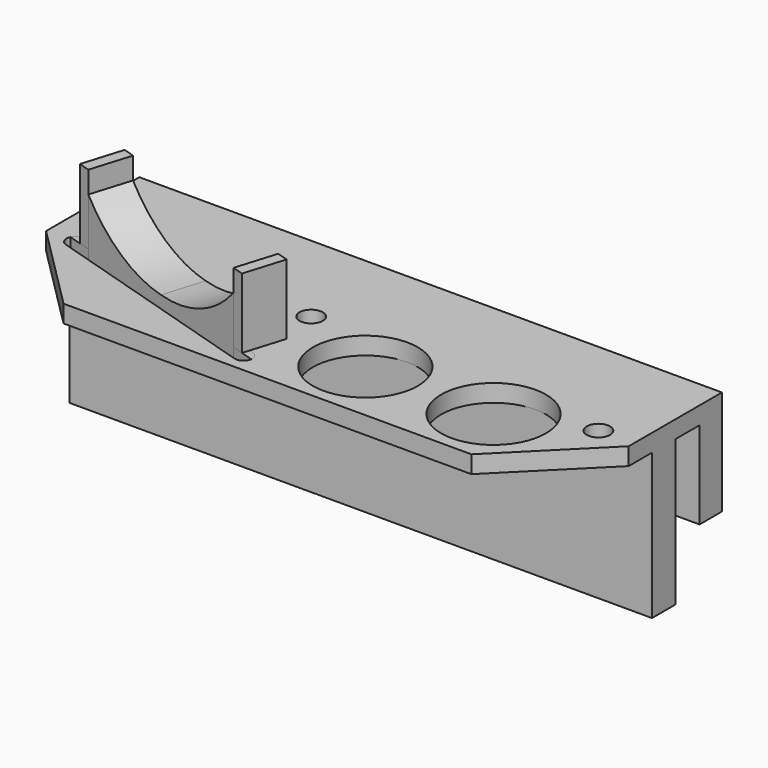
from build123d import *

# Parameters (mm, degrees)
F0_W      = 100
F0_H      = 35
F1_DEPTH  = 3
F2_W      = 100
F2_H      = 5
F3_DEPTH  = 25
F2_H_2    = 4.8
F4_DEPTH  = 15
F5_SIZE   = 15
F6_R      = 9
F6_R_2    = 2
F7_DEPTH  = 30
F9_DEPTH  = 1.25
F10_DEPTH = 6
F12_DEPTH = 3
F14_DEPTH = 12


with BuildPart() as f1:
    # F0 (on Top) → F1 (new body)
    with BuildSketch(Plane.XY):
        Rectangle(F0_W, F0_H)
    extrude(amount=-F1_DEPTH)

    # F2 (on face) → F3 (join)
    with BuildSketch(Plane(origin=(0, 0, -3), x_dir=(1, 0, 0), z_dir=(0, 0, -1))):
        with Locations((0, -5)):
            Rectangle(F2_W, F2_H)
    extrude(amount=F3_DEPTH)

    # F2 (on face) → F4 (join)
    with BuildSketch(Plane(origin=(0, 0, -3), x_dir=(1, 0, 0), z_dir=(0, 0, -1))):
        with Locations((0, -15.1)):
            Rectangle(F2_W, F2_H_2)
    extrude(amount=F4_DEPTH)

    # F5
    f5_edges = [f1.edges().sort_by_distance(p)[0] for p in [
        (50, -17.5, -1.5),
        (-50, -17.5, -1.5),
    ]]
    chamfer(f5_edges, length=F5_SIZE)

    # F6 (on face) → F7 (cut)
    with BuildSketch(Plane.XY):
        with BuildLine():
            Line((-45.4385575571, -3.9344571339), (-7.1863673186, -15.6293253229))
            ThreePointArc((-7.1863673186, -15.6293253229), (-5.3133526275, -14.633425746), (-6.3092522044, -12.760411055))
            Line((-6.3092522044, -12.760411055), (-10.635357075, -11.4377880648))
            Line((-10.635357075, -11.4377880648), (-44.5614424429, -1.0655428661))
            ThreePointArc((-44.5614424429, -1.0655428661), (-46.4344571339, -2.0614424429), (-45.4385575571, -3.9344571339))
        make_face()
        with Locations((30, -6.5)):
            Circle(F6_R)
        with Locations((8, -6.5)):
            Circle(F6_R)
        with Locations((-6.7478097615, 0.3051318111)):
            Circle(F6_R_2)
        with Locations((44, -1.5)):
            Circle(F6_R_2)
    extrude(amount=-F7_DEPTH, mode=Mode.SUBTRACT)


with BuildPart() as f9:
    # F8 (on face) → F9 (new body)
    with BuildSketch(Plane(origin=(-4.1070881898, -13.4336801598, 0), x_dir=(0.956304756, -0.2923717047, 0), z_dir=(-0.2923717047, -0.956304756, 0))):
        Polygon((-5.0527847565, 0), (-22.3027847565, 0), (-39.5527847565, 0), (-39.5527847565, -3), (-5.0527847565, -3), align=None)
        with BuildLine():
            Line((-39.5527847565, 0), (-22.3027847565, 0))
            Line((-22.3027847565, 0), (-5.0527847565, 0))
            Line((-5.0527847565, 0), (-5.0527847565, 8.25))
            ThreePointArc((-5.0527847565, 8.25), (-12.8248807082, 2.4766006665), (-22.3027847565, 0.5))
            ThreePointArc((-22.3027847565, 0.5), (-31.7806888049, 2.4766006665), (-39.5527847565, 8.25))
            Line((-39.5527847565, 8.25), (-39.5527847565, 0))
        make_face()
    extrude(amount=F9_DEPTH)

    # F8 (on face) → F10 (join)
    with BuildSketch(Plane(origin=(-4.1070881898, -13.4336801598, 0), x_dir=(0.956304756, -0.2923717047, 0), z_dir=(-0.2923717047, -0.956304756, 0))):
        with BuildLine():
            Line((-39.5527847565, 0), (-22.3027847565, 0))
            Line((-22.3027847565, 0), (-5.0527847565, 0))
            Line((-5.0527847565, 0), (-5.0527847565, 8.25))
            ThreePointArc((-5.0527847565, 8.25), (-12.8248807082, 2.4766006665), (-22.3027847565, 0.5))
            ThreePointArc((-22.3027847565, 0.5), (-31.7806888049, 2.4766006665), (-39.5527847565, 8.25))
            Line((-39.5527847565, 8.25), (-39.5527847565, 0))
        make_face()
    extrude(amount=-F10_DEPTH)

    # F11 (on face) → F12 (join, through all)
    with BuildSketch(Plane(origin=(0, 0, -3), x_dir=(1, 0, 0), z_dir=(0, 0, -1))):
        with BuildLine():
            ThreePointArc((-46.3413008821, 1.8285002281), (-45.5909842314, 1.1213275813), (-44.5614424429, 1.0655428661))
            Line((-44.5614424429, 1.0655428661), (-41.931604364, 1.869565054))
            Line((-41.931604364, 1.869565054), (-42.2970689949, 3.064945999))
            Line((-42.2970689949, 3.064945999), (-46.3413008821, 1.8285002281))
        make_face()
        with BuildLine():
            Line((-9.3045549142, 13.1517698119), (-8.9390902833, 11.956388867))
            Line((-8.9390902833, 11.956388867), (-6.3092522044, 12.760411055))
            ThreePointArc((-6.3092522044, 12.760411055), (-5.4869177961, 13.3823711418), (-5.260323027, 14.3882155828))
            Line((-5.260323027, 14.3882155828), (-9.3045549142, 13.1517698119))
        make_face()
    extrude(amount=-F12_DEPTH)

    # F13 (on face) → F14 (join)
    with BuildSketch(Plane.XY):
        Polygon((-7.184860055, -6.2185603312), (-9.3045549142, -13.1517698119), (-7.3919454023, -13.7365132214), (-5.272250543, -6.8033037406), align=None)
        Polygon((-44.2096785068, -2.4802025896), (-42.2970689949, -3.064945999), (-40.1773741357, 3.8682634817), (-42.0899836476, 4.4530068912), align=None)
    extrude(amount=F14_DEPTH)


solid = Compound([f1.part, f9.part])
